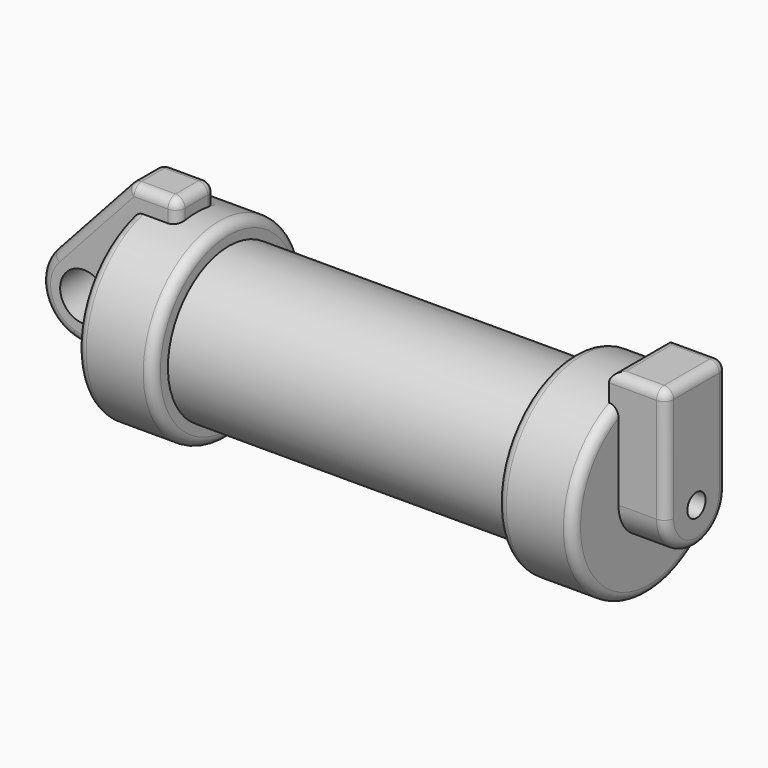
from build123d import *

# Parameters (mm, degrees)
F0_W          = 5.842
F0_H          = 12.7
F0_R          = 3.175
F1_DEPTH      = 3.175
F3_R          = 1.524
F4_DEPTH      = 56.134
F5_DEPTH      = 1.27
F6_DEPTH      = 6.35
F7_R          = 1.27
F8_R          = 1.27
F9_T1_DEPTH   = 12.7
F9_T3_DEPTH   = 12.7
F10_T1_DEPTH  = 4.5187681337
F10_T3_DEPTH  = 3.81
F10_T5_DEPTH  = 14.8458939279
F10_T10_DEPTH = 1.27
F10_T16_DEPTH = 1.27
F10_T20_ANGLE = 89.9999999979
F10_T22_ANGLE = 116.8111069241
F10_T26_DEPTH = 11.6667497034
F10_T31_DEPTH = 4.8482778758
F10_S32_R     = 12.7
F10_T33_DEPTH = 4
F11_T1_DEPTH  = 7.62
F11_T3_DEPTH  = 9.525
F11_T5_DEPTH  = 16.51
F11_T7_DEPTH  = 13.97
F11_S11_W     = 1.27
F11_S11_H     = 1.27
F11_T12_DEPTH = 1.27
F11_S17_W     = 1.27
F11_S17_H     = 1.27
F11_T18_DEPTH = 1.27
F11_S23_W     = 1.27
F11_S23_H     = 1.27
F11_T24_DEPTH = 1.27
F11_T30_DEPTH = 4.8482778758
F11_S31_R     = 12.7
F11_T32_DEPTH = 4
F11_T34_ANGLE = 180


# Not quite as in the source:
# - a fillet or chamfer that OpenCascade refuses, or shapes differently, is made with other operations: its cross-section is extruded or revolved along the edge and cut away or added


with BuildPart() as f1:
    # F0 (on Front) → F1 (new body, symmetric)
    with BuildSketch(Plane.XZ):
        with Locations((2.921, 6.35)):
            Rectangle(F0_W, F0_H)
        with BuildLine():
            Line((-0.9398, 0), (0, 0))
            Line((0, 0), (0, 12.7))
            Line((0, 12.7), (5.842, 12.7))
            Line((5.842, 12.7), (5.842, 15.24))
            Line((5.842, 15.24), (-0.508, 15.24))
            Line((-0.508, 15.24), (-10.8806298187, 3.8475430269))
            ThreePointArc((-10.8806298187, 3.8475430269), (-4.5919612295, 5.3297205562), (-0.9398, 0))
        make_face()
        with BuildLine():
            Line((5.842, 0), (0, 0))
            Line((0, 0), (-0.9398, 0))
            ThreePointArc((-0.9398, 0), (-3.1957909266, -4.5493385486), (-8.1826630726, -5.5069827884))
            Line((-8.1826630726, -5.5069827884), (5.842, -9.398))
            Line((5.842, -9.398), (5.842, 0))
        make_face()
        with BuildLine():
            ThreePointArc((-8.1826630726, -5.5069827884), (-3.1957909266, -4.5493385486), (-0.9398, 0))
            ThreePointArc((-0.9398, 0), (-4.5919612295, 5.3297205562), (-10.8806298187, 3.8475430269))
            ThreePointArc((-10.8806298187, 3.8475430269), (-12.1459778134, -1.5837270034), (-8.1826630726, -5.5069827884))
        make_face()
        with Locations((-6.6548, 0)):
            Circle(F0_R, mode=Mode.SUBTRACT)
    extrude(amount=F1_DEPTH, both=True)

    # F0 (on Front) → F2 (revolve)
    with BuildSketch(Plane.XZ):
        Polygon((5.842, 12.7), (5.842, 0), (66.294, 0), (66.294, 12.7), (56.134, 12.7), (56.134, 10.16), (10.16, 10.16), (10.16, 12.7), align=None)
        with Locations((2.921, 6.35)):
            Rectangle(F0_W, F0_H)
    revolve(axis=Axis((33.147, 0, 0), (-1, 0, 0)))

    # F3 (on face) → F4 (cut, through all)
    with BuildSketch(Plane.YZ.offset(66.294)):
        Circle(F3_R)
    extrude(amount=-F4_DEPTH, mode=Mode.SUBTRACT)

    # F3 (on face) → F5 (join)
    with BuildSketch(Plane.YZ.offset(66.294)):
        with BuildLine():
            ThreePointArc((-5.08, 11.6397422652), (0, 12.7), (5.08, 11.6397422652))
            Line((5.08, 11.6397422652), (5.08, 15.24))
            Line((5.08, 15.24), (-5.08, 15.24))
            Line((-5.08, 15.24), (-5.08, 11.6397422652))
        make_face()
    extrude(amount=-F5_DEPTH)

    # F3 (on face) → F6 (join)
    with BuildSketch(Plane.YZ.offset(66.294)):
        with BuildLine():
            ThreePointArc((-5.08, 0), (0, -5.08), (5.08, 0))
            ThreePointArc((5.08, 0), (0, 5.08), (-5.08, 0))
        make_face()
        Circle(F3_R, mode=Mode.SUBTRACT)
        with BuildLine():
            ThreePointArc((-5.08, 0), (0, 5.08), (5.08, 0))
            Line((5.08, 0), (5.08, 15.24))
            Line((5.08, 15.24), (-5.08, 15.24))
            Line((-5.08, 15.24), (-5.08, 0))
        make_face()
    extrude(amount=F6_DEPTH)

    # F7
    f7_edges = [f1.edges().sort_by_distance(p)[0] for p in [
        (0, 0, -12.7),
        (10.16, 0, -12.7),
        (-4.091332, -3.175, -6.642086),
    ]]
    fillet(f7_edges, radius=F7_R)

    # F8
    f8_edges = [f1.edges().sort_by_distance(p)[0] for p in [
        (56.134, 0, -12.7),
        (66.294, 0, -12.7),
    ]]
    fillet(f8_edges, radius=F8_R)

    # F9: fillet of radius 1.27 on 2 edges, made by hand

    # F9_s2 → F9_t1 (cut)
    with BuildSketch(Plane.XZ.offset(-6.35)):
        with BuildLine():
            ThreePointArc((5.842, 13.97), (5.4700256121, 14.8680256121), (4.572, 15.24))
            Line((4.572, 15.24), (5.842, 15.24))
            Line((5.842, 15.24), (5.842, 13.97))
        make_face()
    extrude(amount=F9_T1_DEPTH, mode=Mode.SUBTRACT)

    # F9_s4 → F9_t3 (cut)
    with BuildSketch(Plane.YZ.offset(-3.683)):
        with BuildLine():
            ThreePointArc((3.175, 13.97), (2.8030256121, 14.8680256121), (1.905, 15.24))
            Line((1.905, 15.24), (3.175, 15.24))
            Line((3.175, 15.24), (3.175, 13.97))
        make_face()
    extrude(amount=F9_T3_DEPTH, mode=Mode.SUBTRACT)

    # F10: fillet of radius 1.27 on 1 edges, made by hand

    # F10_s2 → F10_t1 (cut)
    with BuildSketch(Plane.YZ.offset(0.0532318663)):
        with BuildLine():
            ThreePointArc((-3.175, 13.97), (-2.8030256121, 14.8680256121), (-1.905, 15.24))
            Line((-1.905, 15.24), (-3.175, 15.24))
            Line((-3.175, 15.24), (-3.175, 13.97))
        make_face()
    extrude(amount=F10_T1_DEPTH, mode=Mode.SUBTRACT)

    # F10_s4 → F10_t3 (cut)
    with BuildSketch(Plane.XZ.offset(-1.905)):
        with BuildLine():
            ThreePointArc((-0.8858414267, 14.8250095615), (-0.4601090812, 15.1316286289), (0.0532318663, 15.24))
            Line((0.0532318663, 15.24), (-0.508, 15.24))
            Line((-0.508, 15.24), (-0.8858414267, 14.8250095615))
        make_face()
    extrude(amount=F10_T3_DEPTH, mode=Mode.SUBTRACT)

    # F10_s6 → F10_t5 (cut)
    with BuildSketch(Plane(origin=(6.9785232931, 0, 7.6646451037), x_dir=(0, 1, 0), z_dir=(-0.6732358752, 0, -0.7394277898))):
        with BuildLine():
            ThreePointArc((3.175, -9.3657440555), (2.8030256121, -10.2637696676), (1.905, -10.6357440555))
            Line((1.905, -10.6357440555), (3.175, -10.6357440555))
            Line((3.175, -10.6357440555), (3.175, -9.3657440555))
        make_face()
    extrude(amount=F10_T5_DEPTH, mode=Mode.SUBTRACT)


with BuildPart() as f10_tool8:
    # F10_s9 → F10_t10 (new body)
    with BuildSketch(Plane.XZ.offset(1.905)):
        Polygon((0.0532318663, 13.97), (0.0532318663, 15.24), (-0.508, 15.24), (-0.8858414267, 14.8250095615), align=None)
    extrude(amount=F10_T10_DEPTH)

    # F10_s11 → F10_t12 (revolve, cut)
    with BuildSketch(Plane(origin=(0.0532318663, -1.905, 13.97), x_dir=(0.4042054705, 0, -0.9146682118), z_dir=(-0.9146682118, 0, -0.4042054705))):
        with BuildLine():
            ThreePointArc((0, -1.27), (1.27, 0), (0, 1.27))
            Line((0, 1.27), (0, -1.27))
        make_face()
    revolve(axis=Axis((0.0532318663, -1.905, 13.97), (0, -1, 0)), mode=Mode.SUBTRACT)


with BuildPart() as f1_1:
    add(f1.part)

    # F10_t7: cut F10_tool8
    add(f10_tool8.part, mode=Mode.SUBTRACT)


with BuildPart() as f10_tool14:
    # F10_s15 → F10_t16 (new body)
    with BuildSketch(Plane.XZ.offset(-1.905)):
        Polygon((0.0532318663, 13.97), (0.0532318663, 15.24), (-0.508, 15.24), (-0.8858414267, 14.8250095615), align=None)
    extrude(amount=-F10_T16_DEPTH)

    # F10_s17 → F10_t18 (revolve, cut)
    with BuildSketch(Plane(origin=(0.0532318663, 1.905, 13.97), x_dir=(0.4042054705, 0, -0.9146682118), z_dir=(0.9146682118, 0, 0.4042054705))):
        with BuildLine():
            ThreePointArc((0, -1.27), (1.27, 0), (0, 1.27))
            Line((0, 1.27), (0, -1.27))
        make_face()
    revolve(axis=Axis((0.0532318663, 1.905, 13.97), (0, 1, 0)), mode=Mode.SUBTRACT)


with BuildPart() as f1_2:
    add(f1_1.part)

    # F10_t13: cut F10_tool14
    add(f10_tool14.part, mode=Mode.SUBTRACT)

    # F10_s19 → F10_t20 (revolve, cut)
    with BuildSketch(Plane.YZ.offset(4.572)):
        with BuildLine():
            ThreePointArc((-3.175, 13.97), (-2.8030256121, 14.8680256121), (-1.905, 15.24))
            Line((-1.905, 15.24), (-3.175, 15.24))
            Line((-3.175, 15.24), (-3.175, 13.97))
        make_face()
    revolve(axis=Axis((4.572, -3.175, 13.97), (0, 1, 0)), revolution_arc=F10_T20_ANGLE, mode=Mode.SUBTRACT)

    # F10_s21 → F10_t22 (revolve, cut)
    with BuildSketch(Plane(origin=(-3.0162650989, 0, -3.3128214309), x_dir=(0, 1, 0), z_dir=(0.6732358752, 0, 0.7394277898))):
        with BuildLine():
            ThreePointArc((3.175, 9.3657440555), (2.8030256121, 10.2637696676), (1.905, 10.6357440555))
            Line((1.905, 10.6357440555), (3.175, 10.6357440555))
            Line((3.175, 10.6357440555), (3.175, 9.3657440555))
        make_face()
    revolve(axis=Axis((-6.6548, 3.175, 0), (0, -1, 0)), revolution_arc=F10_T22_ANGLE, mode=Mode.SUBTRACT)


with BuildPart() as f10_tool24:
    # F10_s25 → F10_t26 (new body)
    with BuildSketch(Plane(origin=(-6.179167626, 0, 1.7143547379), x_dir=(0, 1, 0), z_dir=(0.9636015378, 0, -0.2673426199))):
        with BuildLine():
            ThreePointArc((3.175, -6.2241116667), (2.8030256121, -7.1221372788), (1.905, -7.4941116667))
            Line((1.905, -7.4941116667), (3.175, -7.4941116667))
            Line((3.175, -7.4941116667), (3.175, -6.2241116667))
        make_face()
    extrude(amount=F10_T26_DEPTH)

    split(bisect_by=Plane.YZ, keep=Keep.BOTTOM)


with BuildPart() as f1_3:
    add(f1_2.part)

    # F10_t23: cut F10_tool24
    add(f10_tool24.part, mode=Mode.SUBTRACT)


with BuildPart() as f10_tool29:
    # F10_s30 → F10_t31 (new body)
    with BuildSketch(Plane.XY.offset(9.1217221242)):
        with BuildLine():
            ThreePointArc((5.842, -1.905), (5.4700256121, -2.8030256121), (4.572, -3.175))
            Line((4.572, -3.175), (5.842, -3.175))
            Line((5.842, -3.175), (5.842, -1.905))
        make_face()
    extrude(amount=F10_T31_DEPTH)

    # F10_s32 → F10_t33 (cut, symmetric)
    with BuildSketch(Plane.YZ.offset(5.2)):
        Circle(F10_S32_R)
    extrude(amount=F10_T33_DEPTH, both=True, mode=Mode.SUBTRACT)


with BuildPart() as f1_4:
    add(f1_3.part)

    # F10_t28: cut F10_tool29
    add(f10_tool29.part, mode=Mode.SUBTRACT)

    # F11: fillet of radius 1.27 on 8 edges, made by hand

    # F11_s2 → F11_t1 (cut)
    with BuildSketch(Plane.XZ.offset(-3.81)):
        with BuildLine():
            ThreePointArc((71.374, 15.24), (72.2720256121, 14.8680256121), (72.644, 13.97))
            Line((72.644, 13.97), (72.644, 15.24))
            Line((72.644, 15.24), (71.374, 15.24))
        make_face()
    extrude(amount=F11_T1_DEPTH, mode=Mode.SUBTRACT)

    # F11_s4 → F11_t3 (cut)
    with BuildSketch(Plane.YZ.offset(61.849)):
        with BuildLine():
            ThreePointArc((-3.81, 15.24), (-4.7080256121, 14.8680256121), (-5.08, 13.97))
            Line((-5.08, 13.97), (-5.08, 15.24))
            Line((-5.08, 15.24), (-3.81, 15.24))
        make_face()
        with BuildLine():
            ThreePointArc((5.08, 13.97), (4.7080256121, 14.8680256121), (3.81, 15.24))
            Line((3.81, 15.24), (5.08, 15.24))
            Line((5.08, 15.24), (5.08, 13.97))
        make_face()
    extrude(amount=F11_T3_DEPTH, mode=Mode.SUBTRACT)

    # F11_s6 → F11_t5 (cut)
    with BuildSketch(Plane.XZ.offset(-8.255)):
        with BuildLine():
            ThreePointArc((65.024, 13.97), (65.3959743879, 14.8680256121), (66.294, 15.24))
            Line((66.294, 15.24), (65.024, 15.24))
            Line((65.024, 15.24), (65.024, 13.97))
        make_face()
    extrude(amount=F11_T5_DEPTH, mode=Mode.SUBTRACT)

    # F11_s8 → F11_t7 (cut)
    with BuildSketch(Plane.XY):
        with BuildLine():
            ThreePointArc((71.374, -5.08), (72.2720256121, -4.7080256121), (72.644, -3.81))
            Line((72.644, -3.81), (72.644, -5.08))
            Line((72.644, -5.08), (71.374, -5.08))
        make_face()
        with BuildLine():
            ThreePointArc((71.374, 5.08), (72.2720256121, 4.7080256121), (72.644, 3.81))
            Line((72.644, 3.81), (72.644, 5.08))
            Line((72.644, 5.08), (71.374, 5.08))
        make_face()
    extrude(amount=F11_T7_DEPTH, mode=Mode.SUBTRACT)


with BuildPart() as f11_tool10:
    # F11_s11 → F11_t12 (new body)
    with BuildSketch(Plane.YZ.offset(4.572)):
        with Locations((2.54, 14.605)):
            Rectangle(F11_S11_W, F11_S11_H)
    extrude(amount=F11_T12_DEPTH)

    # F11_s13 → F11_t14 (revolve, cut)
    with BuildSketch(Plane(origin=(4.572, 1.905, 13.97), x_dir=(0, -0.7071067812, -0.7071067812), z_dir=(0, -0.7071067812, 0.7071067812))):
        with BuildLine():
            ThreePointArc((0, -1.27), (1.27, 0), (0, 1.27))
            Line((0, 1.27), (0, -1.27))
        make_face()
    revolve(axis=Axis((4.572, 1.905, 13.97), (1, 0, 0)), mode=Mode.SUBTRACT)


with BuildPart() as f1_5:
    add(f1_4.part)

    # F11_t9: cut F11_tool10
    add(f11_tool10.part, mode=Mode.SUBTRACT)


with BuildPart() as f11_tool16:
    # F11_s17 → F11_t18 (new body)
    with BuildSketch(Plane.XZ.offset(-3.81)):
        with Locations((72.009, 14.605)):
            Rectangle(F11_S17_W, F11_S17_H)
    extrude(amount=-F11_T18_DEPTH)

    # F11_s19 → F11_t20 (revolve, cut)
    with BuildSketch(Plane(origin=(71.374, 3.81, 13.97), x_dir=(-0.7071067812, 0, -0.7071067812), z_dir=(0.7071067812, 0, -0.7071067812))):
        with BuildLine():
            ThreePointArc((0, -1.27), (1.27, 0), (0, 1.27))
            Line((0, 1.27), (0, -1.27))
        make_face()
    revolve(axis=Axis((71.374, 3.81, 13.97), (0, 1, 0)), mode=Mode.SUBTRACT)


with BuildPart() as f1_6:
    add(f1_5.part)

    # F11_t15: cut F11_tool16
    add(f11_tool16.part, mode=Mode.SUBTRACT)


with BuildPart() as f11_tool22:
    # F11_s23 → F11_t24 (new body)
    with BuildSketch(Plane.XY.offset(13.97)):
        with Locations((72.009, -4.445)):
            Rectangle(F11_S23_W, F11_S23_H)
    extrude(amount=F11_T24_DEPTH)

    # F11_s25 → F11_t26 (revolve, cut)
    with BuildSketch(Plane(origin=(71.374, -3.81, 13.97), x_dir=(-0.7071067812, 0.7071067812, 0), z_dir=(0.7071067812, 0.7071067812, 0))):
        with BuildLine():
            ThreePointArc((0, -1.27), (1.27, 0), (0, 1.27))
            Line((0, 1.27), (0, -1.27))
        make_face()
    revolve(axis=Axis((71.374, -3.81, 13.97), (0, 0, 1)), mode=Mode.SUBTRACT)


with BuildPart() as f1_7:
    add(f1_6.part)

    # F11_t21: cut F11_tool22
    add(f11_tool22.part, mode=Mode.SUBTRACT)


with BuildPart() as f11_tool28:
    # F11_s29 → F11_t30 (new body)
    with BuildSketch(Plane.XY.offset(9.1217221242)):
        with BuildLine():
            ThreePointArc((5.842, 1.905), (5.4700256121, 2.8030256121), (4.572, 3.175))
            Line((4.572, 3.175), (5.842, 3.175))
            Line((5.842, 3.175), (5.842, 1.905))
        make_face()
    extrude(amount=F11_T30_DEPTH)

    # F11_s31 → F11_t32 (cut, symmetric)
    with BuildSketch(Plane.YZ.offset(5.2)):
        Circle(F11_S31_R)
    extrude(amount=F11_T32_DEPTH, both=True, mode=Mode.SUBTRACT)


with BuildPart() as f1_8:
    add(f1_7.part)

    # F11_t27: cut F11_tool28
    add(f11_tool28.part, mode=Mode.SUBTRACT)

    # F11_s33 → F11_t34 (revolve, cut)
    with BuildSketch(Plane.XY):
        with BuildLine():
            ThreePointArc((71.374, -5.08), (72.2720256121, -4.7080256121), (72.644, -3.81))
            Line((72.644, -3.81), (72.644, -5.08))
            Line((72.644, -5.08), (71.374, -5.08))
        make_face()
    revolve(axis=Axis((72.644, 0, 0), (1, 0, 0)), revolution_arc=F11_T34_ANGLE, mode=Mode.SUBTRACT)


solid = f1_8.part
